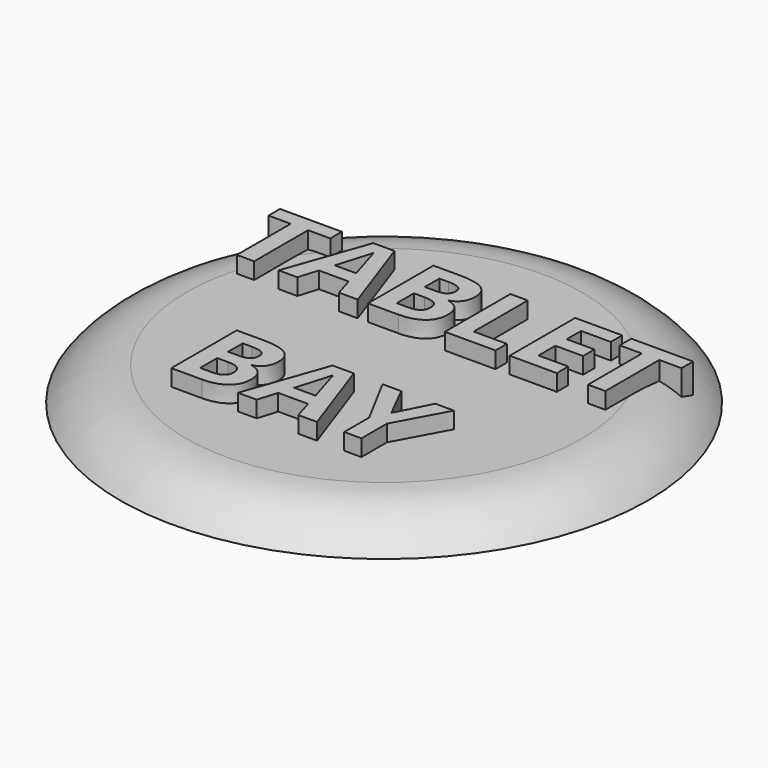
from build123d import *

# Parameters (mm, degrees)
F0_R          = 16
F1_DEPTH      = 2
F3_TEXT_SIZE  = 6.9444444444
F4_DEPTH      = 1
F4_DEPTH_BACK = 1


# Not quite as in the source:
# - a fillet or chamfer that OpenCascade refuses, or shapes differently, is made with other operations: its cross-section is extruded or revolved along the edge and cut away or added
# - Text() gives the source's letters only with a copy of the font that has no kerning and outlines rounded to 1/6400 em; it was checked with that copy


with BuildPart() as f1:
    # F0 (on Top) → F1 (new body)
    with BuildSketch(Plane.XY):
        Circle(F0_R)
    extrude(amount=F1_DEPTH)

    # F2: fillet of radius 5 on 1 edges, made by hand

    # F2_s1 → F2_t2 (revolve, cut)
    with BuildSketch(Plane.XZ):
        with BuildLine():
            ThreePointArc((16, 0), (14.2360679775, 1.472135955), (12, 2))
            Line((12, 2), (16, 2))
            Line((16, 2), (16, 0))
        make_face()
    revolve(axis=Axis((0, 0, 2), (0, 0, 1)), mode=Mode.SUBTRACT)

    # F3 (on face) → F4 (join, two sides)
    with BuildSketch(Plane.XY.offset(2)) as f4_sk:
        with Locations((-12.8119574653, 3)):
            Text('TABLET', F3_TEXT_SIZE, font='Open Sans', font_style=FontStyle.BOLD, text_align=(TextAlign.LEFT, TextAlign.BOTTOM))
        with Locations((-7.1207682292, -8)):
            Text('BAY', F3_TEXT_SIZE, font='Open Sans', font_style=FontStyle.BOLD, text_align=(TextAlign.LEFT, TextAlign.BOTTOM))
    extrude(amount=F4_DEPTH)
    extrude(f4_sk.sketch, amount=-F4_DEPTH_BACK)


solid = f1.part
